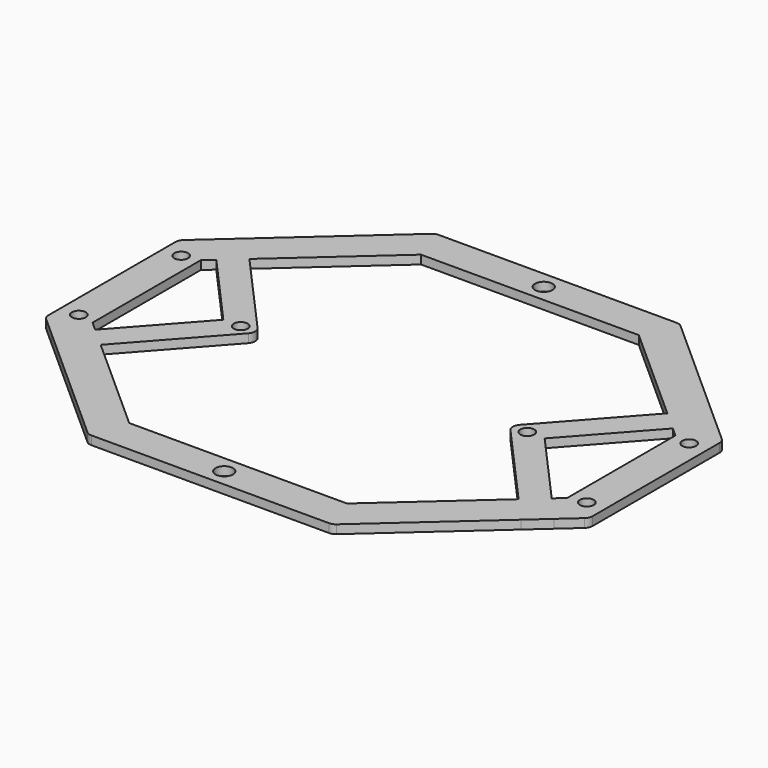
from build123d import *

# Parameters (mm, degrees)
F0_R     = 1
F0_R_2   = 0.8
F1_DEPTH = 1
F2_R     = 1


with BuildPart() as f1:
    # F0 (on Top) → F1 (new body)
    with BuildSketch(Plane.XY):
        Polygon((14.0690184001, 25), (0, 25), (-14.0690184001, 25), (-26.7296075576, 13.6899425008), (-24.0647631939, 10.7068896154), (-12.5425545984, 21), (0, 21), (12.5425545984, 21), (24.0647631939, 10.7068896154), (26.7296075576, 13.6899425008), align=None)
        with Locations((0, 23)):
            Circle(F0_R, mode=Mode.SUBTRACT)
        Polygon((28.9542586869, 11.7025995837), (26.7296075576, 13.6899425008), (24.0647631939, 10.7068896154), (26.2894143232, 8.7195466983), align=None)
        Polygon((-24.0647631939, 10.7068896154), (-26.7296075576, 13.6899425008), (-28.9542586869, 11.7025995837), (-26.2894143232, 8.7195466983), align=None)
        Polygon((31.3294992745, 9.5807309025), (28.9542586869, 11.7025995837), (26.2894143232, 8.7195466983), (27.3294992745, 7.7904097951), (27.3294992745, 0.0814010352), (27.3294992745, -0.0814010352), (27.3294992745, -7.7904097951), (26.2894143232, -8.7195466983), (28.9542586869, -11.7025995837), (31.3294992745, -9.5807309025), (31.3294992745, 0), align=None)
        with Locations((29.25, -7.3612159322)):
            Circle(F0_R_2, mode=Mode.SUBTRACT)
        with Locations((29.25, 7.3612159322)):
            Circle(F0_R_2, mode=Mode.SUBTRACT)
        Polygon((26.2894143232, 8.7195466983), (24.0647631939, 10.7068896154), (14.5, 0), (24.0647631939, -10.7068896154), (26.2894143232, -8.7195466983), (18.5, 0), align=None)
        with Locations((16.5, 0)):
            Circle(F0_R_2, mode=Mode.SUBTRACT)
        Polygon((-26.2894143232, 8.7195466983), (-28.9542586869, 11.7025995837), (-31.3294992745, 9.5807309025), (-31.3294992745, 0), (-31.3294992745, -9.5807309025), (-28.9542586869, -11.7025995837), (-26.2894143232, -8.7195466983), (-27.3294992745, -7.7904097951), (-27.3294992745, -0.0814010352), (-27.3294992745, 0.0814010352), (-27.3294992745, 7.7904097951), align=None)
        with Locations((-29.25, -7.3612159322)):
            Circle(F0_R_2, mode=Mode.SUBTRACT)
        with Locations((-29.25, 7.3612159322)):
            Circle(F0_R_2, mode=Mode.SUBTRACT)
        Polygon((-14.5, 0), (-24.0647631939, 10.7068896154), (-26.2894143232, 8.7195466983), (-18.5, 0), (-26.2894143232, -8.7195466983), (-24.0647631939, -10.7068896154), align=None)
        with Locations((-16.5, 0)):
            Circle(F0_R_2, mode=Mode.SUBTRACT)
        Polygon((26.2894143232, -8.7195466983), (24.0647631939, -10.7068896154), (26.7296075576, -13.6899425008), (28.9542586869, -11.7025995837), align=None)
        Polygon((26.7296075576, -13.6899425008), (24.0647631939, -10.7068896154), (12.5425545984, -21), (0, -21), (-12.5425545984, -21), (-24.0647631939, -10.7068896154), (-26.7296075576, -13.6899425008), (-14.0690184001, -25), (0, -25), (14.0690184001, -25), align=None)
        with Locations((0, -23)):
            Circle(F0_R, mode=Mode.SUBTRACT)
        Polygon((-26.7296075576, -13.6899425008), (-24.0647631939, -10.7068896154), (-26.2894143232, -8.7195466983), (-28.9542586869, -11.7025995837), align=None)
    extrude(amount=F1_DEPTH)

    # F2
    f2_edges = [f1.edges().sort_by_distance(p)[0] for p in [
        (-14.069018, 25, 0.5),
        (-31.329499, 9.580731, 0.5),
        (-31.329499, -9.580731, 0.5),
        (-14.069018, -25, 0.5),
        (14.069018, -25, 0.5),
        (31.329499, -9.580731, 0.5),
        (31.329499, 9.580731, 0.5),
        (14.069018, 25, 0.5),
        (14.5, 0, 0.5),
        (-14.5, 0, 0.5),
    ]]
    fillet(f2_edges, radius=F2_R)


solid = f1.part
